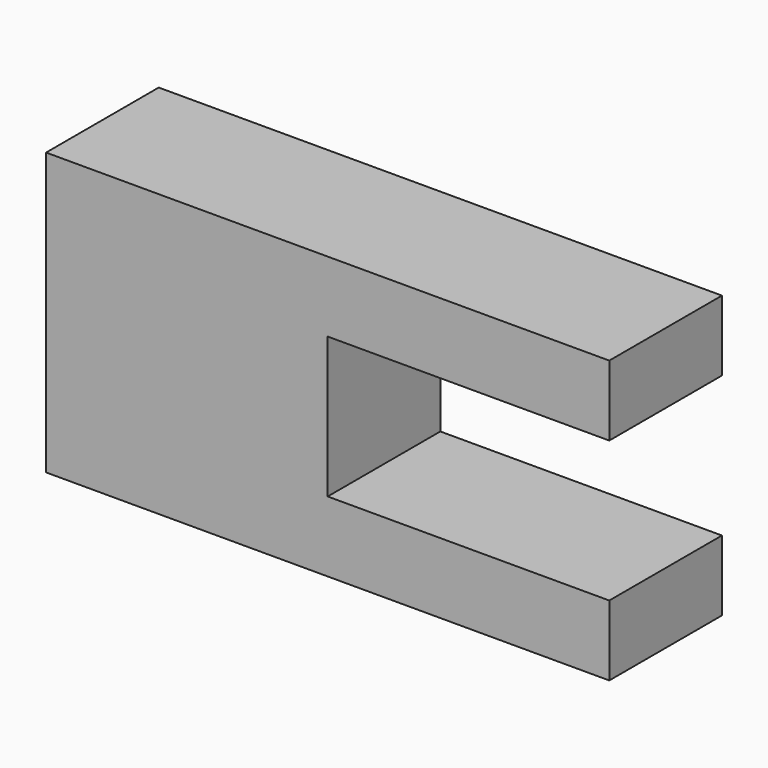
from build123d import *

# Parameters (mm, degrees)
F0_W     = 101.6
F0_H     = 50.8
F1_DEPTH = 25.4
F2_W     = 50.8
F2_H     = 25.4
F3_DEPTH = 130
F4_DEPTH = 25.401


# Not quite as in the source:
# - an extrude ends at something that could not be found from the text; its depth is read off the source's solid


with BuildPart() as f1:
    # F0 (on Front) → F1 (new body)
    with BuildSketch(Plane.XZ):
        Rectangle(F0_W, F0_H)
    extrude(amount=F1_DEPTH)

    # F2 (on Front) → F3 (cut, through all)
    with BuildSketch(Plane.XZ):
        with Locations((25.4, 0)):
            Rectangle(F2_W, F2_H)
    extrude(amount=-F3_DEPTH, mode=Mode.SUBTRACT)

    # F2 (on Front) → F4 (cut, through all)
    with BuildSketch(Plane.XZ):
        with Locations((25.4, 0)):
            Rectangle(F2_W, F2_H)
    extrude(amount=F4_DEPTH, mode=Mode.SUBTRACT)


solid = f1.part
